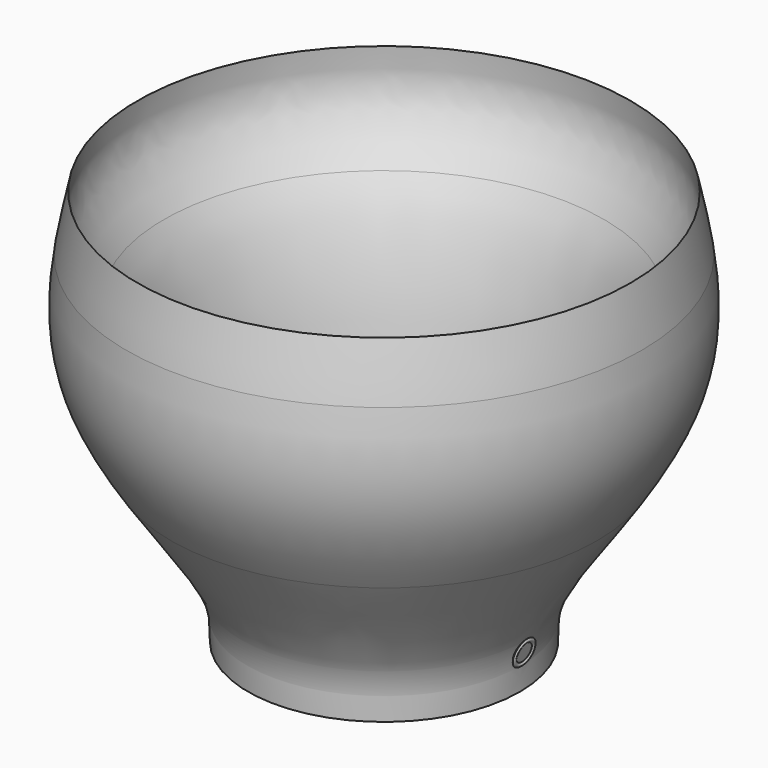
from build123d import *


with BuildPart() as f1:
    # F0 (on Front) → F1 (revolve)
    with BuildSketch(Plane.XZ):
        with BuildLine():
            add(Edge.make_bspline(
                [(19.6823217034, -6.6014872209), (18.7206290933, -7.4863491309), (17.5676079465, -8.5412161557), (16.6606779031, -9.2215613008), (16.5172192351, -9.3254513944)],
                knots=[0, 0, 0, 0, 0.5821747808, 0.6959078834, 0.6959078834, 0.6959078834, 0.6959078834], degree=3))
            add(Edge.make_bspline(
                [(23.7838823749, 10.1932772593), (24.2970848929, 6.840613956), (24.4178453084, 1.3242383799), (21.093212182, -4.4477596725), (19.6823217034, -6.6014872209)],
                knots=[0.1255407693, 0.1255407693, 0.1255407693, 0.1255407693, 0.3707684145, 0.5266538311, 0.5266538311, 0.5266538311, 0.5266538311], degree=3))
            add(Edge.make_bspline(
                [(23.7838823557, 10.1932772629), (22.5530164904, 9.153802728), (21.3274805944, 8.1001474), (20.3086007386, 6.497125607)],
                knots=[0.0071128484, 0.0071128484, 0.0071128484, 0.0071128484, 0.27405021, 0.27405021, 0.27405021, 0.27405021], degree=3))
            add(Edge.make_bspline(
                [(20.3086007386, 6.497125607), (18.9438893572, 4.3500009258), (17.4757524028, -0.2772106808), (16.8935087075, -4.7649402342), (16.755240937, -6.2066463042)],
                knots=[0.27405021, 0.27405021, 0.27405021, 0.27405021, 0.6315923221, 0.8021612393, 0.8021612393, 0.8021612393, 0.8021612393], degree=3))
            add(Edge.make_bspline(
                [(16.755240937, -6.2066463042), (16.6552314343, -7.2494367288), (16.5812677523, -8.2881791115), (16.5172192351, -9.3254513944)],
                knots=[0.8021612393, 0.8021612393, 0.8021612393, 0.8021612393, 0.9255342605, 0.9255342605, 0.9255342605, 0.9255342605], degree=3))
        make_face()
        with BuildLine():
            add(Edge.make_bspline(
                [(19.6823217034, -6.6014872209), (17.4171980587, -10.0592036547), (12.5537292031, -16.1629021911), (12.5385838339, -19.5460692495), (12.5492885709, -21.20067738)],
                knots=[0.5266538311, 0.5266538311, 0.5266538311, 0.5266538311, 0.7769211256, 1, 1, 1, 1], degree=3))
            add(Edge.make_bspline(
                [(19.6823217034, -6.6014872209), (18.7206290933, -7.4863491309), (17.5676079465, -8.5412161557), (16.6606779031, -9.2215613008), (16.5172192351, -9.3254513944)],
                knots=[0, 0, 0, 0, 0.5821747808, 0.6959078834, 0.6959078834, 0.6959078834, 0.6959078834], degree=3))
            add(Edge.make_bspline(
                [(16.5172192351, -9.3254513944), (16.1336488497, -9.6032259185), (15.7841216901, -9.8288168601), (15.4340223068, -10.0539055119)],
                knots=[0.6959078834, 0.6959078834, 0.6959078834, 0.6959078834, 1, 1, 1, 1], degree=3))
            add(Edge.make_bspline(
                [(15.4340223068, -10.0539055119), (15.2801119472, -10.3720102908), (14.1971702129, -12.3893155375), (11.3362161193, -15.3503692976), (9.1659848619, -15.7282313026), (8.3738614299, -15.7529823482)],
                knots=[0.281908143, 0.281908143, 0.281908143, 0.281908143, 0.3519178239, 0.7265638945, 0.9449180046, 0.9449180046, 0.9449180046, 0.9449180046], degree=3))
            add(Edge.make_bspline(
                [(8.3738614299, -15.7529823482), (8.1740404178, -15.7592260456), (7.9746646983, -15.7581908421), (7.7750007622, -15.7529823482)],
                knots=[0.9449180046, 0.9449180046, 0.9449180046, 0.9449180046, 1, 1, 1, 1], degree=3))
            Line((7.7750007622, -15.7529823482), (0.5906730657, -15.7529823482))
            add(Edge.make_bspline(
                [(10.4511072859, -21.20067738), (9.6412763004, -20.3488201147), (8.0167557876, -18.6399949078), (5.2456073558, -16.1032388951), (2.2052839685, -15.8744723638), (0.5906730657, -15.7529823482)],
                knots=[0, 0, 0, 0, 0.3179359251, 0.6377792914, 1, 1, 1, 1], degree=3))
            Line((10.4511072859, -21.20067738), (12.5492885709, -21.20067738))
        make_face()
        with BuildLine():
            add(Edge.make_bspline(
                [(23.7838823557, 10.1932772629), (22.5530164904, 9.153802728), (21.3274805944, 8.1001474), (20.3086007386, 6.497125607)],
                knots=[0.0071128484, 0.0071128484, 0.0071128484, 0.0071128484, 0.27405021, 0.27405021, 0.27405021, 0.27405021], degree=3))
            add(Edge.make_bspline(
                [(22.7640811354, 15.3368497267), (23.1432789035, 13.6207649594), (23.5211557201, 11.9096250621), (23.7838823749, 10.1932772593)],
                knots=[0, 0, 0, 0, 0.1255407693, 0.1255407693, 0.1255407693, 0.1255407693], degree=3))
            add(Edge.make_bspline(
                [(22.7640811354, 15.3368497267), (22.9201033117, 14.065351127), (23.2625710046, 11.2744197209), (21.3498954205, 8.1811543908), (20.3086007386, 6.497125607)],
                knots=[0, 0, 0, 0, 0.4555821748, 1, 1, 1, 1], degree=3))
        make_face()
        with BuildLine():
            add(Edge.make_bspline(
                [(16.5172192351, -9.3254513944), (16.1336488497, -9.6032259185), (15.7841216901, -9.8288168601), (15.4340223068, -10.0539055119)],
                knots=[0.6959078834, 0.6959078834, 0.6959078834, 0.6959078834, 1, 1, 1, 1], degree=3))
            add(Edge.make_bspline(
                [(16.755240937, -6.2066463042), (16.6552314343, -7.2494367288), (16.5812677523, -8.2881791115), (16.5172192351, -9.3254513944)],
                knots=[0.8021612393, 0.8021612393, 0.8021612393, 0.8021612393, 0.9255342605, 0.9255342605, 0.9255342605, 0.9255342605], degree=3))
            add(Edge.make_bspline(
                [(16.755240937, -6.2066463042), (16.4044399801, -7.4841944835), (16.053773505, -8.7729922694), (15.4340223068, -10.0539055119)],
                knots=[0, 0, 0, 0, 0.281908143, 0.281908143, 0.281908143, 0.281908143], degree=3))
        make_face()
    revolve(axis=Axis((0, 0, 5.9850515099), (0, 0, -1)))

    # F2 (on Front) → F3 (revolve)
    with BuildSketch(Plane.XZ):
        with BuildLine():
            add(Edge.make_bspline(
                [(12.7333556769, -18.7082347352), (12.7740238366, -18.7907127998), (12.8548636625, -18.9546620031), (12.7076612214, -19.0581256067), (12.634512037, -19.1095396876)],
                knots=[0, 0, 0, 0, 0.5030708471, 1, 1, 1, 1], degree=3))
            Line((12.7333556769, -18.7082347352), (12.634512037, -19.1095396876))
        make_face()
        with BuildLine():
            add(Edge.make_bspline(
                [(12.4912384255, -17.7732517499), (12.4659192386, -17.9335036999), (12.4138150114, -18.2632853804), (12.6248629774, -18.5571623933), (12.7333556769, -18.7082347352)],
                knots=[0, 0, 0, 0, 0.4859334508, 1, 1, 1, 1], degree=3))
            Line((12.7333556769, -18.7082347352), (12.9366270456, -17.8829534421))
            Line((12.9366270456, -17.8829534421), (12.4912384255, -17.7732517499))
        make_face()
        with BuildLine():
            Line((12.634512037, -19.1095396876), (12.7333556769, -18.7082347352))
            add(Edge.make_bspline(
                [(12.4912384255, -17.7732517499), (12.4659192386, -17.9335036999), (12.4138150114, -18.2632853804), (12.6248629774, -18.5571623933), (12.7333556769, -18.7082347352)],
                knots=[0, 0, 0, 0, 0.4859334508, 1, 1, 1, 1], degree=3))
            Line((12.4912384255, -17.7732517499), (12.3356003172, -17.7349172189))
            add(Edge.make_bspline(
                [(12.634512037, -19.1095396876), (12.4763407595, -18.8037343288), (12.2830712375, -18.0616036857), (12.3185150717, -17.8224569612), (12.3356003172, -17.7349172189)],
                knots=[0, 0, 0, 0, 0.6517513838, 1, 1, 1, 1], degree=3))
        make_face()
    revolve(axis=Axis((12.9386744507, 0, -17.8834577293), (-0.97098068, 0, 0.2391579373)))


solid = f1.part
